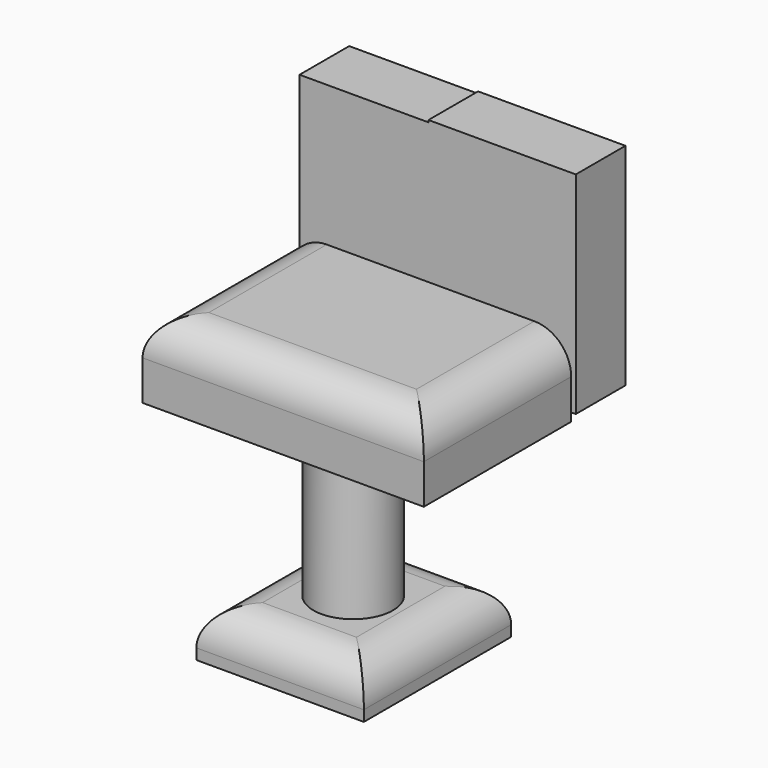
from build123d import *

# Parameters (mm, degrees)
F0_W         = 38.7927275151
F0_H         = 10.5539034121
F1_DEPTH     = 25.4
F2_W         = 8.5572190583
F2_H         = 29.094544705
F3_DEPTH     = 20.32
F4_W         = 8.5572199896
F4_H         = 28.5240663216
F5_DEPTH     = 17.78
F6_R         = 5.4792946357
F7_DEPTH     = 27.94
F8_W         = 23.1044916436
F8_H         = 6.5605361015
F9_DEPTH     = 25.4
F10_T1_DEPTH = 64.1927275151
F10_T3_DEPTH = 38.1
F10_T5_DEPTH = 48.5044916436
F10_T7_DEPTH = 50.8


# Not quite as in the source:
# - a fillet or chamfer that OpenCascade refuses, or shapes differently, is made with other operations: its cross-section is extruded or revolved along the edge and cut away or added


with BuildPart() as f1:
    # F0 (on Front) → F1 (new body)
    with BuildSketch(Plane.XZ):
        with Locations((0.2852408215, -0.2852405887)):
            Rectangle(F0_W, F0_H)
    extrude(amount=F1_DEPTH)

    # F2 (on Right) → F3 (join)
    with BuildSketch(Plane.YZ):
        with Locations((4.2786095291, 10.1260424126)):
            Rectangle(F2_W, F2_H)
    extrude(amount=F3_DEPTH)

    # F4 (on Right) → F5 (join)
    with BuildSketch(Plane.YZ):
        with Locations((4.2786099948, 10.1260435767)):
            Rectangle(F4_W, F4_H)
    extrude(amount=-F5_DEPTH)

    # F6 (on Top) → F7 (join)
    with BuildSketch(Plane.XY):
        with Locations((0, -12.9784494638)):
            Circle(F6_R)
    extrude(amount=-F7_DEPTH)

    # F8 (on Front) → F9 (join)
    with BuildSketch(Plane.XZ):
        with Locations((-0.1426204108, -31.0912309214)):
            Rectangle(F8_W, F8_H)
    extrude(amount=F9_DEPTH)

    # F10: fillet of radius 5.08 on 7 edges, made by hand

    # F10_s2 → F10_t1 (cut)
    with BuildSketch(Plane.YZ.offset(-31.811122936)):
        with BuildLine():
            ThreePointArc((-20.32, 4.9917111173), (-23.9121024484, 3.5038135658), (-25.4, -0.0882888827))
            Line((-25.4, -0.0882888827), (-25.4, 4.9917111173))
            Line((-25.4, 4.9917111173), (-20.32, 4.9917111173))
        make_face()
    extrude(amount=F10_T1_DEPTH, mode=Mode.SUBTRACT)

    # F10_s4 → F10_t3 (cut)
    with BuildSketch(Plane.XZ):
        with BuildLine():
            ThreePointArc((-14.031122936, 4.9917111173), (-17.6232253844, 3.5038135658), (-19.111122936, -0.0882888827))
            Line((-19.111122936, -0.0882888827), (-19.111122936, 4.9917111173))
            Line((-19.111122936, 4.9917111173), (-14.031122936, 4.9917111173))
        make_face()
        with BuildLine():
            ThreePointArc((14.6016045791, 4.9917111173), (18.1937070275, 3.5038135658), (19.6816045791, -0.0882888827))
            Line((19.6816045791, -0.0882888827), (19.6816045791, 4.9917111173))
            Line((19.6816045791, 4.9917111173), (14.6016045791, 4.9917111173))
        make_face()
    extrude(amount=F10_T3_DEPTH, mode=Mode.SUBTRACT)

    # F10_s6 → F10_t5 (cut)
    with BuildSketch(Plane.YZ.offset(-24.3948662326)):
        with BuildLine():
            ThreePointArc((-20.32, -27.8109628707), (-23.9121024484, -29.2988604223), (-25.4, -32.8909628707))
            Line((-25.4, -32.8909628707), (-25.4, -27.8109628707))
            Line((-25.4, -27.8109628707), (-20.32, -27.8109628707))
        make_face()
        with BuildLine():
            ThreePointArc((-5.08, -27.8109628707), (-1.4878975516, -29.2988604223), (0, -32.8909628707))
            Line((0, -32.8909628707), (0, -27.8109628707))
            Line((0, -27.8109628707), (-5.08, -27.8109628707))
        make_face()
    extrude(amount=F10_T5_DEPTH, mode=Mode.SUBTRACT)

    # F10_s8 → F10_t7 (cut)
    with BuildSketch(Plane.XZ.offset(-12.7)):
        with BuildLine():
            ThreePointArc((6.329625411, -27.8109628707), (9.9217278595, -29.2988604223), (11.409625411, -32.8909628707))
            Line((11.409625411, -32.8909628707), (11.409625411, -27.8109628707))
            Line((11.409625411, -27.8109628707), (6.329625411, -27.8109628707))
        make_face()
        with BuildLine():
            ThreePointArc((-6.6148662326, -27.8109628707), (-10.206968681, -29.2988604223), (-11.6948662326, -32.8909628707))
            Line((-11.6948662326, -32.8909628707), (-11.6948662326, -27.8109628707))
            Line((-11.6948662326, -27.8109628707), (-6.6148662326, -27.8109628707))
        make_face()
    extrude(amount=F10_T7_DEPTH, mode=Mode.SUBTRACT)


solid = f1.part
